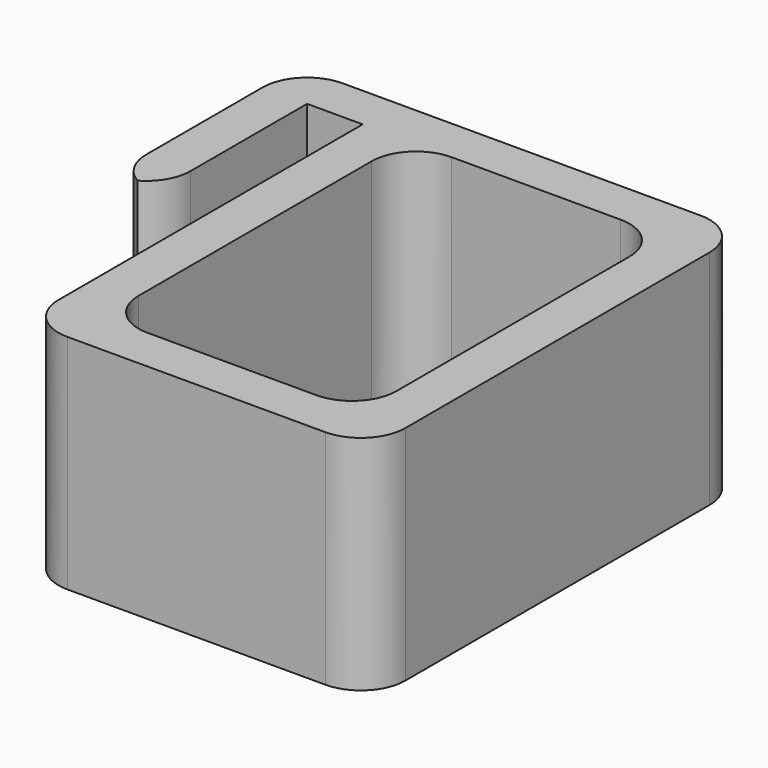
from build123d import *

# Parameters (mm, degrees)
F0_W        = 29.464
F0_H        = 43.434
F1_DEPTH    = 25.4
F2_T1_DEPTH = 50.8
F3_R        = 5.08


# Not quite as in the source:
# - a fillet or chamfer that OpenCascade refuses, or shapes differently, is made with other operations: its cross-section is extruded or revolved along the edge and cut away or added


with BuildPart() as f1:
    # F0 (on Top) → F1 (new body)
    with BuildSketch(Plane.XY):
        Polygon((25.527, -26.797), (25.527, 26.797), (-25.527, 26.797), (-25.527, 0), (-20.447, 0), (-20.447, 21.717), (-14.097, 21.717), (-14.097, -26.797), align=None)
        with Locations((5.715, 0)):
            Rectangle(F0_W, F0_H, mode=Mode.SUBTRACT)
    extrude(amount=F1_DEPTH)

    # F2: fillet of radius 5.08 on 6 edges, made by hand

    # F2_s2 → F2_t1 (cut)
    with BuildSketch(Plane.XY.offset(-12.7)):
        with BuildLine():
            ThreePointArc((-20.447, 26.797), (-24.0391024484, 25.3091024484), (-25.527, 21.717))
            Line((-25.527, 21.717), (-25.527, 26.797))
            Line((-25.527, 26.797), (-20.447, 26.797))
        make_face()
        with BuildLine():
            ThreePointArc((25.527, 21.717), (24.0391024484, 25.3091024484), (20.447, 26.797))
            Line((20.447, 26.797), (25.527, 26.797))
            Line((25.527, 26.797), (25.527, 21.717))
        make_face()
        with BuildLine():
            ThreePointArc((-9.017, -26.797), (-12.6091024484, -25.3091024484), (-14.097, -21.717))
            Line((-14.097, -21.717), (-14.097, -26.797))
            Line((-14.097, -26.797), (-9.017, -26.797))
        make_face()
        with BuildLine():
            ThreePointArc((20.447, -26.797), (24.0391024484, -25.3091024484), (25.527, -21.717))
            Line((25.527, -21.717), (25.527, -26.797))
            Line((25.527, -26.797), (20.447, -26.797))
        make_face()
        with BuildLine():
            ThreePointArc((-25.527, 0), (-21.9348975516, 1.4878975516), (-20.447, 5.08))
            Line((-20.447, 5.08), (-20.447, 0))
            Line((-20.447, 0), (-25.527, 0))
        make_face()
        with BuildLine():
            ThreePointArc((-25.527, 5.08), (-24.0391024484, 1.4878975516), (-20.447, 0))
            Line((-20.447, 0), (-25.527, 0))
            Line((-25.527, 0), (-25.527, 5.08))
        make_face()
    extrude(amount=F2_T1_DEPTH, mode=Mode.SUBTRACT)

    # F3
    f3_edges = [f1.edges().sort_by_distance(p)[0] for p in [
        (-9.017, -21.717, 12.7),
        (20.447, -21.717, 12.7),
        (20.447, 21.717, 12.7),
        (-9.017, 21.717, 12.7),
    ]]
    fillet(f3_edges, radius=F3_R)


solid = f1.part
